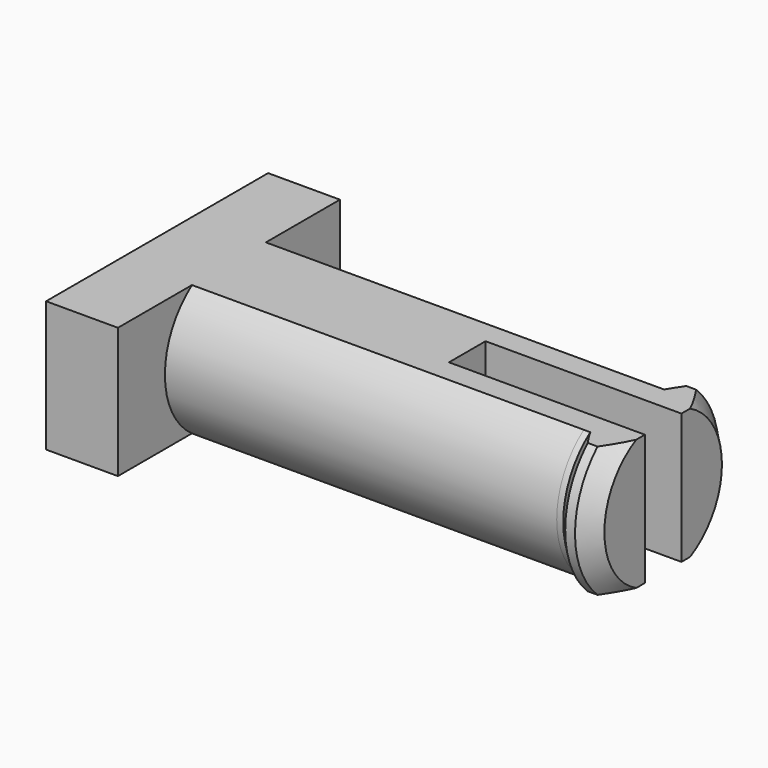
from build123d import *

# Parameters (mm, degrees)
F3_W         = 38.5
F3_H         = 34
F3_W_2       = 8.5
F3_H_2       = 4
F4_DEPTH     = 15.501
F5_T4_ANGLE  = 146.9201983829
F5_S5_R      = 2.45
F5_T6_DEPTH  = 4
F5_T10_ANGLE = 146.9201983829
F5_S11_R     = 2.45
F5_T12_DEPTH = 4
F5_T14_ANGLE = 146.9201983829
F5_T16_ANGLE = 146.9201983829
F6_W         = 6
F6_H         = 1.4
F7_DEPTH     = 4.001


# Not quite as in the source:
# - a fillet or chamfer that OpenCascade refuses, or shapes differently, is made with other operations: its cross-section is extruded or revolved along the edge and cut away or added


with BuildPart() as f2:
    # F1 (on Front) → F2 (revolve)
    with BuildSketch(Plane.XZ):
        Polygon((0, 7.5), (0, 0), (15.5, 0), (15.5, 2.75), (14.2, 2.75), (14.2, 2.45), (2.2, 2.45), (2.2, 7.5), align=None)
    revolve(axis=Axis((8.8834212145, 0, 0), (1, 0, 0)))

    # F3 (on Right) → F4 (cut, through all)
    with BuildSketch(Plane.YZ):
        Rectangle(F3_W, F3_H)
        Rectangle(F3_W_2, F3_H_2, mode=Mode.SUBTRACT)
    extrude(amount=F4_DEPTH, mode=Mode.SUBTRACT)

    # F5: chamfer of 0.5 on 4 edges, made by hand


with BuildPart() as f5_tool2:
    # F5_s3 → F5_t4 (revolve)
    with BuildSketch(Plane(origin=(0, 0, 0), x_dir=(1, 0, 0), z_dir=(0, -0.958621714, -0.2846829983))):
        Polygon((14.2, -2.25), (14.7, -2.75), (14.2, -2.75), align=None)
    revolve(axis=Axis((14.2, 0, 0), (1, 0, 0)), revolution_arc=F5_T4_ANGLE)

    # F5_s5 → F5_t6 (cut, symmetric)
    with BuildSketch(Plane.YZ.offset(14.4)):
        Circle(F5_S5_R)
    extrude(amount=F5_T6_DEPTH, both=True, mode=Mode.SUBTRACT)


with BuildPart() as f2_1:
    add(f2.part)

    # F5_t1: cut F5_tool2
    add(f5_tool2.part, mode=Mode.SUBTRACT)


with BuildPart() as f5_tool8:
    # F5_s9 → F5_t10 (revolve)
    with BuildSketch(Plane(origin=(0, 0, 0), x_dir=(1, 0, 0), z_dir=(0, 0.958621714, 0.2846829983))):
        Polygon((14.7, -2.75), (14.2, -2.25), (14.2, -2.75), align=None)
    revolve(axis=Axis((14.2, 0, 0), (1, 0, 0)), revolution_arc=F5_T10_ANGLE)

    # F5_s11 → F5_t12 (cut, symmetric)
    with BuildSketch(Plane.YZ.offset(14.4)):
        Circle(F5_S11_R)
    extrude(amount=F5_T12_DEPTH, both=True, mode=Mode.SUBTRACT)


with BuildPart() as f2_2:
    add(f2_1.part)

    # F5_t7: cut F5_tool8
    add(f5_tool8.part, mode=Mode.SUBTRACT)

    # F5_s13 → F5_t14 (revolve, cut)
    with BuildSketch(Plane(origin=(0, 0, 0), x_dir=(1, 0, 0), z_dir=(0, -0.958621714, -0.2846829983))):
        Polygon((15, -2.75), (15.5, -2.25), (15.5, -2.75), align=None)
    revolve(axis=Axis((15.5, 0, 0), (1, 0, 0)), revolution_arc=F5_T14_ANGLE, mode=Mode.SUBTRACT)

    # F5_s15 → F5_t16 (revolve, cut)
    with BuildSketch(Plane(origin=(0, 0, 0), x_dir=(1, 0, 0), z_dir=(0, 0.958621714, 0.2846829983))):
        Polygon((15.5, -2.25), (15, -2.75), (15.5, -2.75), align=None)
    revolve(axis=Axis((15.5, 0, 0), (1, 0, 0)), revolution_arc=F5_T16_ANGLE, mode=Mode.SUBTRACT)

    # F6 (on face) → F7 (cut, through all)
    with BuildSketch(Plane.XY.offset(2)):
        with Locations((12.5, 0)):
            Rectangle(F6_W, F6_H)
    extrude(amount=-F7_DEPTH, mode=Mode.SUBTRACT)


solid = f2_2.part
